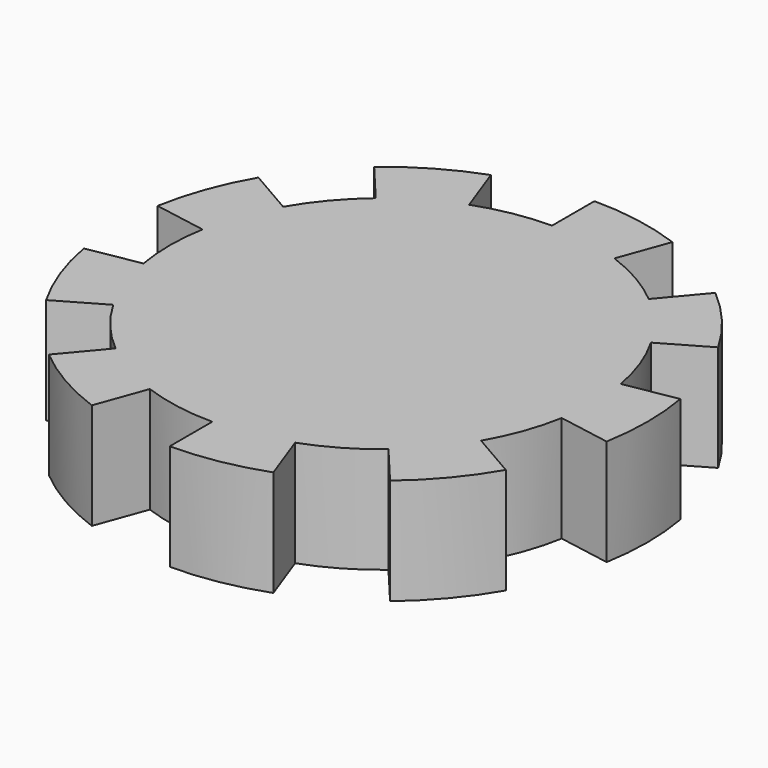
from build123d import *

# Parameters (mm, degrees)
F0_R            = 10
F1_DEPTH        = 4
F3_DEPTH        = 4.001
F3_COPIES_COUNT = 9


# Not quite as in the source:
# - a pattern or mirror of a feature is missing from the dataset's text; its kind, count and spacing are read off the source's solid


with BuildPart() as f1:
    # F0 (on Top) → F1 (new body)
    with BuildSketch(Plane.XY):
        Circle(F0_R)
    extrude(amount=F1_DEPTH)

    # F2 (on face) → F3 (cut, through all)
    with BuildSketch(Plane.XY.offset(4)):
        with BuildLine():
            ThreePointArc((-2.7361611466, 7.5175409663), (-1.3891854213, 7.8784620241), (0, 8))
            Line((0, 8), (0, 10))
            ThreePointArc((0, 10), (-1.7364817767, 9.8480775301), (-3.4202014333, 9.3969262079))
            Line((-3.4202014333, 9.3969262079), (-2.7361611466, 7.5175409663))
        make_face()
    f3 = extrude(amount=-F3_DEPTH, mode=Mode.SUBTRACT)

    # F3_copies: F3 ×9 about axis
    f3_copies_axis = Axis((0, 0, 0), (0, 0, 1))
    for i in range(1, F3_COPIES_COUNT):
        add(f3.rotate(f3_copies_axis, i * 360 / F3_COPIES_COUNT), mode=Mode.SUBTRACT)


solid = f1.part
